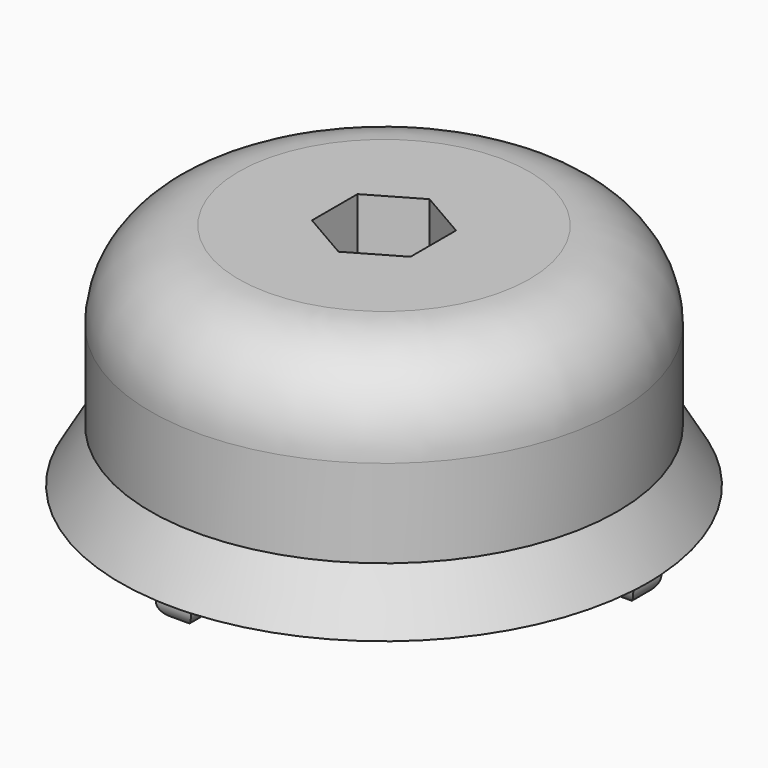
from build123d import *

# Parameters (mm, degrees)
F0_R     = 15
F1_DEPTH = 3
F1_TAPER = 30
F2_DEPTH = 10
F4_DEPTH = 3
F5_R     = 1.5
F6_DEPTH = 10.001
F7_W     = 13.4332590942
F7_H     = 2
F7_W_2   = 2
F7_H_2   = 13.4332590942
F8_DEPTH = 1
F9_R     = 0.99999
F10_R    = 5


# Not quite as in the source:
# - a fillet or chamfer is up to 0.001 mm smaller than in the source, because OpenCascade refuses the exact size


with BuildPart() as f1:
    # F0 (on Top) → F1 (new body)
    with BuildSketch(Plane.XY):
        Circle(F0_R)
    extrude(amount=F1_DEPTH, taper=F1_TAPER)

    # F2 (add): a face of the model
    f2_faces = [f1.faces().sort_by_distance(p)[0] for p in [
        (0, 0, 3),
    ]]
    extrude(f2_faces, amount=F2_DEPTH)

    # F3 (on face) → F4 (cut)
    with BuildSketch(Plane.XY.offset(13)):
        Polygon((2.8, -1.6165807537), (2.8, 1.6165807537), (0, 3.2331615075), (-2.8, 1.6165807537), (-2.8, -1.6165807537), (0, -3.2331615075), align=None)
    extrude(amount=-F4_DEPTH, mode=Mode.SUBTRACT)

    # F5 (on face) → F6 (cut, through all)
    with BuildSketch(Plane.XY.offset(10)):
        Circle(F5_R)
    extrude(amount=-F6_DEPTH, mode=Mode.SUBTRACT)

    # F7 (on face) → F8 (join)
    with BuildSketch(Plane(origin=(0, 0, 0), x_dir=(1, 0, 0), z_dir=(0, 0, -1))):
        with Locations((-8.25, 0)):
            Rectangle(F7_W, F7_H)
        with Locations((0, 8.25)):
            Rectangle(F7_W_2, F7_H_2)
        with Locations((8.25, 0)):
            Rectangle(F7_W, F7_H)
        with Locations((0, -8.25)):
            Rectangle(F7_W_2, F7_H_2)
    extrude(amount=F8_DEPTH)

    # F9 (radius 1 in the source; OpenCascade refuses exactly that, so slightly less here)
    f9_edges = [f1.edges().sort_by_distance(p)[0] for p in [
        (-1, 8.25, -1),
        (1, 8.25, -1),
        (8.25, 1, -1),
        (14.96663, 0, -1),
        (8.25, -1, -1),
        (1.53337, 0, -1),
        (-8.25, 1, -1),
        (-8.25, -1, -1),
        (1, -8.25, -1),
        (-1, -8.25, -1),
        (0, 14.96663, -1),
        (0, 1.53337, -1),
        (0, -1.53337, -1),
        (-1.53337, 0, -1),
        (-14.96663, 0, -1),
        (0, -14.96663, -1),
    ]]
    fillet(f9_edges, radius=F9_R)

    # F10
    f10_edges = [f1.edges().sort_by_distance(p)[0] for p in [
        (-13.267949, 0, 13),
    ]]
    fillet(f10_edges, radius=F10_R)


solid = f1.part
